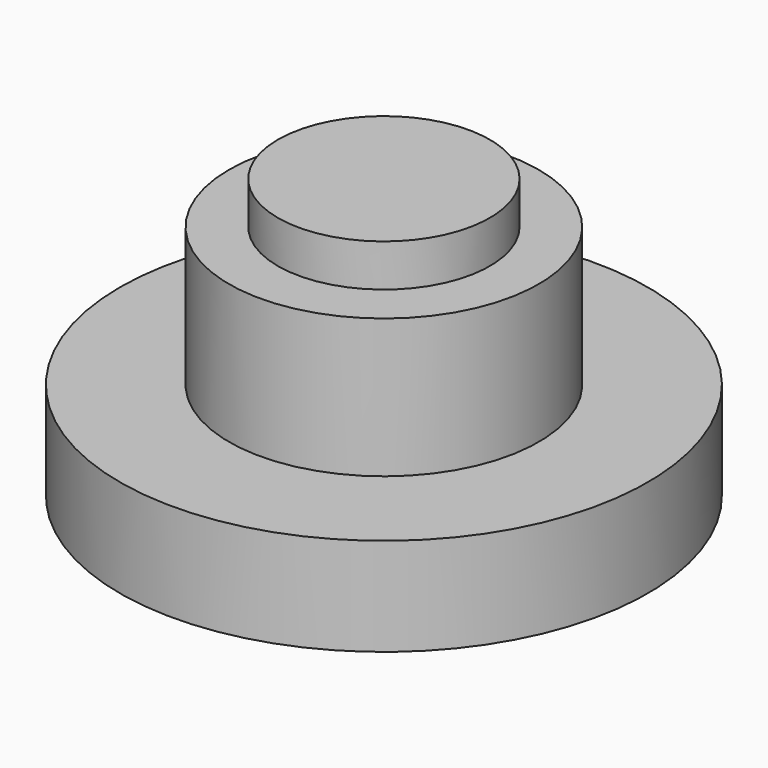
from build123d import *

# Parameters (mm, degrees)
F0_W = 0.25
F0_H = 2


# Not quite as in the source:
# - a feature names something its author has since deleted; it is built from what else it names


with BuildPart() as f1:
    # F0 (on Front) → F1 (revolve)
    with BuildSketch(Plane.XZ):
        Polygon((0, 2.2599502219), (0, 5.5599502219), (-3.25, 5.5599502219), (-3.25, 4.2599502219), (-4.75, 4.2599502219), (-4.75, 0), (-2.75, 0), (-2.75, 2.2599502219), align=None)
    revolve(axis=Axis((0, 0, 3.9099502219), (0, 0, 1)))


with BuildPart() as f2:
    # F0 (on Front) → F2 (revolve)
    with BuildSketch(Plane.XZ):
        with Locations((-6.7192060259, -2)):
            Rectangle(F0_W, F0_H)
        with Locations((-5.4692060259, -2)):
            Rectangle(F0_W, F0_H)
        with Locations((-4.2192060259, -2)):
            Rectangle(F0_W, F0_H)
        Polygon((0, -1), (0, 2.2599502219), (-2.75, 2.2599502219), (-2.75, 0), (-4.75, 0), (-6.2268639432, 0), (-8.0942060259, 0), (-8.0942060259, -3), (-7.8442060259, -3), (-7.8442060259, -1), (-6.8442060259, -1), (-6.5942060259, -1), (-5.5942060259, -1), (-5.3442060259, -1), (-4.3442060259, -1), (-4.0942060259, -1), (-3.0942060259, -1), (-2.8442060259, -1), (-1.8442060259, -1), (-1.5942060259, -1), align=None)
    revolve(axis=Axis((0, 0, 0.6299751109), (0, 0, 1)))


solid = Compound([f1.part, f2.part])
